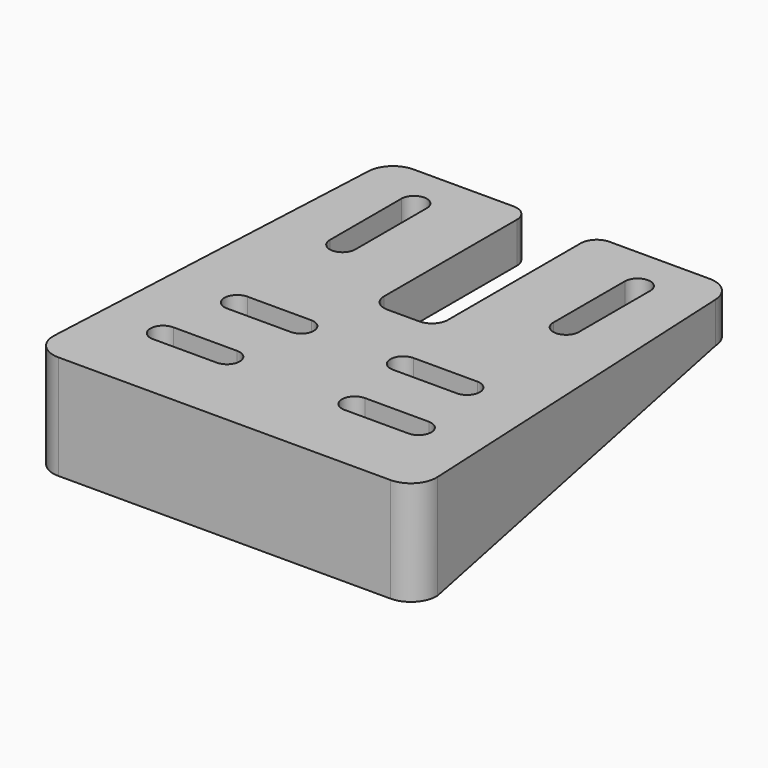
from build123d import *

# Parameters (mm, degrees)
F1_DEPTH = 6.35
F3_DEPTH = 10
F4_SIZE2 = 9.99999
F4_SIZE  = 57.99999
F5_SIZE2 = 9.99999
F5_SIZE  = 57.99999


# Not quite as in the source:
# - a fillet or chamfer is up to 0.001 mm smaller than in the source, because OpenCascade refuses the exact size


with BuildPart() as f1:
    # F0 (on Top) → F1 (new body)
    with BuildSketch(Plane.XY):
        with BuildLine():
            Line((-26.0047037435, 0), (0, 0))
            Line((0, 0), (26.0047037435, 0))
            ThreePointArc((26.0047037435, 0), (28.9008830765, 1.2409883525), (30, 4.1939273644))
            Line((30, 4.1939273644), (27.1847426542, 62.1939273644))
            ThreePointArc((27.1847426542, 62.1939273644), (25.9484580453, 64.896179333), (23.1894463977, 66))
            Line((23.1894463977, 66), (7.5, 66))
            ThreePointArc((7.5, 66), (5.732233047, 65.267766953), (5, 63.5))
            Line((5, 63.5), (5, 37.5))
            ThreePointArc((5, 37.5), (4.267766953, 35.732233047), (2.5, 35))
            Line((2.5, 35), (0, 35))
            Line((0, 35), (-2.5, 35))
            ThreePointArc((-2.5, 35), (-4.267766953, 35.732233047), (-5, 37.5))
            Line((-5, 37.5), (-5, 63.5))
            ThreePointArc((-5, 63.5), (-5.732233047, 65.267766953), (-7.5, 66))
            Line((-7.5, 66), (-23.1894463977, 66))
            ThreePointArc((-23.1894463977, 66), (-25.9484580453, 64.896179333), (-27.1847426542, 62.1939273644))
            Line((-27.1847426542, 62.1939273644), (-30, 4.1939273644))
            ThreePointArc((-30, 4.1939273644), (-28.9008830765, 1.2409883525), (-26.0047037435, 0))
        make_face()
        with BuildLine():
            ThreePointArc((-20, 11), (-22, 13), (-20, 15))
            Line((-20, 15), (-10, 15))
            ThreePointArc((-10, 15), (-8, 13), (-10, 11))
            Line((-10, 11), (-20, 11))
        make_face(mode=Mode.SUBTRACT)
        with BuildLine():
            Line((-18, 27), (-8, 27))
            ThreePointArc((-8, 27), (-6, 25), (-8, 23))
            Line((-8, 23), (-18, 23))
            ThreePointArc((-18, 23), (-20, 25), (-18, 27))
        make_face(mode=Mode.SUBTRACT)
        with BuildLine():
            Line((10, 15), (20, 15))
            ThreePointArc((20, 15), (22, 13), (20, 11))
            Line((20, 11), (10, 11))
            ThreePointArc((10, 11), (8, 13), (10, 15))
        make_face(mode=Mode.SUBTRACT)
        with BuildLine():
            Line((18, 23), (8, 23))
            ThreePointArc((8, 23), (6, 25), (8, 27))
            Line((8, 27), (18, 27))
            ThreePointArc((18, 27), (20, 25), (18, 23))
        make_face(mode=Mode.SUBTRACT)
        with BuildLine():
            ThreePointArc((-15.5, 45), (-17.5, 43), (-19.5, 45))
            Line((-19.5, 45), (-19.5, 59))
            ThreePointArc((-19.5, 59), (-17.5, 61), (-15.5, 59))
            Line((-15.5, 59), (-15.5, 45))
        make_face(mode=Mode.SUBTRACT)
        with BuildLine():
            Line((15.5, 45), (15.5, 59))
            ThreePointArc((15.5, 59), (17.5, 61), (19.5, 59))
            Line((19.5, 59), (19.5, 45))
            ThreePointArc((19.5, 45), (17.5, 43), (15.5, 45))
        make_face(mode=Mode.SUBTRACT)
    extrude(amount=F1_DEPTH)

    # F2 (on face) → F3 (join)
    with BuildSketch(Plane.XY):
        with BuildLine():
            ThreePointArc((26.0047037435, 0), (28.9008830765, 1.2409883525), (30, 4.1939273644))
            Line((30, 4.1939273644), (26.0047037435, 4))
            Line((26.0047037435, 4), (-26.0047037435, 4))
            Line((-26.0047037435, 4), (-30, 4.1939273644))
            ThreePointArc((-30, 4.1939273644), (-28.9008830765, 1.2409883525), (-26.0047037435, 0))
            Line((-26.0047037435, 0), (0, 0))
            Line((0, 0), (26.0047037435, 0))
        make_face()
        Polygon((-30, 4.1939273644), (-26.0047037435, 4), (-23.1894463977, 62), (-27.1847426542, 62.1939273644), align=None)
        Polygon((26.0047037435, 4), (30, 4.1939273644), (27.1847426542, 62.1939273644), (23.1894463977, 62), align=None)
    extrude(amount=-F3_DEPTH)

    # F4 (size 58 and 10 in the source; OpenCascade refuses exactly that, so slightly less here)
    f4_edges = [f1.edges().sort_by_distance(p)[0] for p in [
        (-25.187095, 62.096964, -10),
    ]]
    f4_side = f1.faces().sort_by_distance((0, 0.864246, -10))[0]
    chamfer(f4_edges, length=F4_SIZE, length2=F4_SIZE2, reference=f4_side)

    # F5 (size 58 and 10 in the source; OpenCascade refuses exactly that, so slightly less here)
    f5_edges = [f1.edges().sort_by_distance(p)[0] for p in [
        (25.187095, 62.096964, -10),
    ]]
    f5_side = f1.faces().sort_by_distance((-25.139818, 3.992207, -10))[0]
    chamfer(f5_edges, length=F5_SIZE, length2=F5_SIZE2, reference=f5_side)


solid = f1.part
